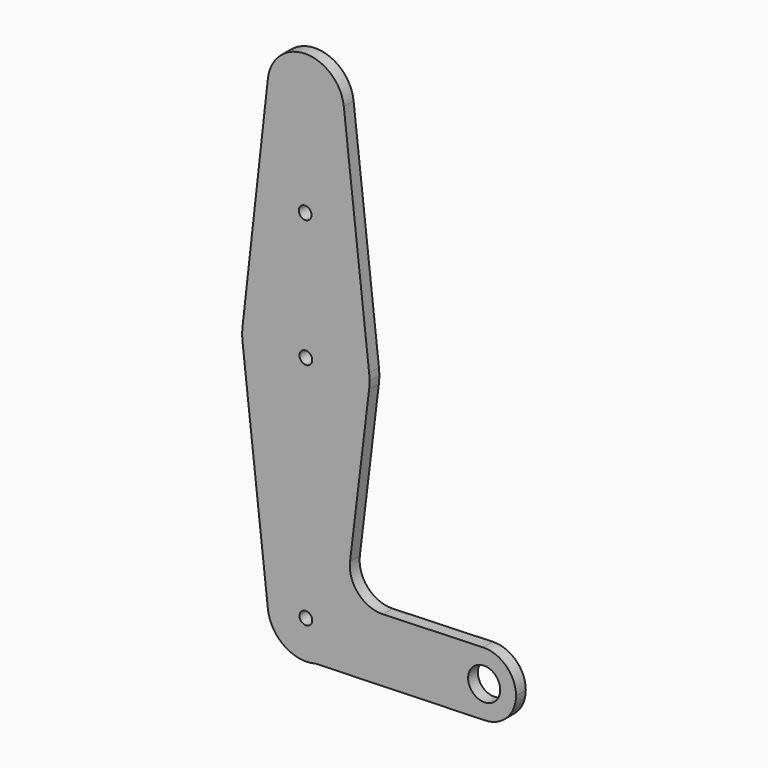
from build123d import *

# Parameters (mm, degrees)
F0_R     = 1.5875
F0_R_2   = 4.002551
F1_DEPTH = 3.048


# Not quite as in the source:
# - ends of sketch curves that miss each other by under 0.0002 mm in the source are joined


with BuildPart() as f1:
    # F0 (on Front) → F1 (new body)
    with BuildSketch(Plane.XZ):
        with BuildLine():
            ThreePointArc((-49.358992, 68.087074), (-40.422958, 57.518497), (-30.367971, 67.028741))
            ThreePointArc((-30.367971, 67.028741), (-30.382727, 67.558729), (-30.426949, 68.087075))
            ThreePointArc((-30.426949, 68.087075), (-39.892971, 76.553741), (-49.358992, 68.087074))
        make_face()
        with BuildLine():
            ThreePointArc((-30.426949, 68.087075), (-30.382727, 67.558729), (-30.367971, 67.028741))
            ThreePointArc((-30.367971, 67.028741), (-40.422958, 57.518497), (-49.358992, 68.087074))
            Line((-49.358992, 68.087074), (-55.669672, 11.642631))
            ThreePointArc((-55.669672, 11.642631), (-39.892971, 25.753741), (-24.116269, 11.642631))
            Line((-24.116269, 11.642631), (-30.426949, 68.087075))
        make_face()
        with Locations((-40.057853, 41.628741)):
            Circle(F0_R, mode=Mode.SUBTRACT)
        with BuildLine():
            ThreePointArc((-24.017971, 9.878741), (-24.042564, 10.762054), (-24.116269, 11.642631))
            ThreePointArc((-24.116269, 11.642631), (-39.892971, 25.753741), (-55.669672, 11.642631))
            ThreePointArc((-55.669672, 11.642631), (-55.767971, 9.878741), (-55.669672, 8.114851))
            ThreePointArc((-55.669672, 8.114851), (-39.963754, -5.996101), (-24.132626, 7.974232))
            ThreePointArc((-24.132626, 7.974232), (-24.04666, 8.924762), (-24.017971, 9.878741))
        make_face()
        with Locations((-39.892971, 9.878741)):
            Circle(F0_R, mode=Mode.SUBTRACT)
        with BuildLine():
            ThreePointArc((-24.132626, 7.974232), (-39.963754, -5.996101), (-55.669672, 8.114851))
            Line((-55.669672, 8.114851), (-49.358989, -48.329593))
            ThreePointArc((-49.358989, -48.329593), (-40.422958, -37.761015), (-30.367971, -47.271259))
            ThreePointArc((-30.367971, -47.271259), (-32.349953, -53.087487), (-37.471069, -56.483209))
            Line((-37.471069, -56.483209), (4.796929, -55.205133))
            ThreePointArc((4.796929, -55.205133), (-3.376393, -47.525644), (4.28816, -39.338314))
            Line((4.28816, -39.338314), (-20.714858, -40.185732))
            ThreePointArc((-20.714858, -40.185732), (-26.843275, -37.613772), (-28.876937, -31.286317))
            Line((-28.876937, -31.286317), (-24.132626, 7.974232))
        make_face()
        with BuildLine():
            ThreePointArc((-30.367971, -47.271259), (-40.422958, -37.761015), (-49.358992, -48.329593))
            ThreePointArc((-49.358992, -48.329593), (-46.909184, -53.713182), (-41.753864, -56.61271))
            Line((-41.753864, -56.61271), (-37.471069, -56.483209))
            ThreePointArc((-37.471069, -56.483209), (-32.349953, -53.087487), (-30.367971, -47.271259))
        make_face()
        with Locations((-39.892971, -47.271259)):
            Circle(F0_R, mode=Mode.SUBTRACT)
        with BuildLine():
            Line((-37.471069, -56.483209), (-41.753864, -56.61271))
            ThreePointArc((-41.753864, -56.61271), (-39.60509, -56.791908), (-37.471069, -56.483209))
        make_face()
        with BuildLine():
            ThreePointArc((12.494529, -47.271259), (10.073811, -41.564331), (4.28816, -39.338314))
            ThreePointArc((4.28816, -39.338314), (-3.376393, -47.525644), (4.796929, -55.205133))
            ThreePointArc((4.796929, -55.205133), (10.253876, -52.798451), (12.494529, -47.271259))
        make_face()
        with Locations((4.557029, -47.271259)):
            Circle(F0_R_2, mode=Mode.SUBTRACT)
    extrude(amount=F1_DEPTH)


solid = f1.part
